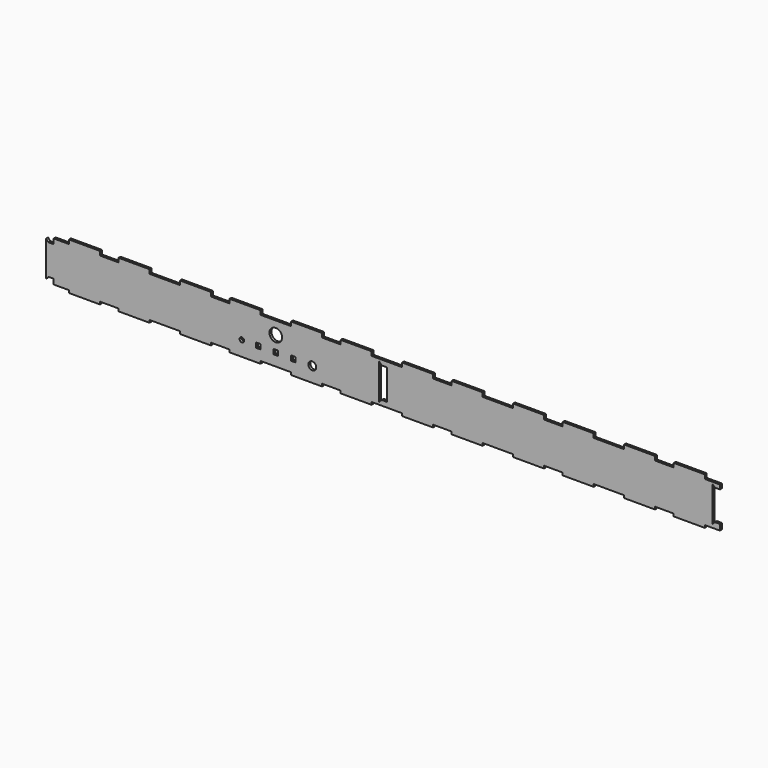
from build123d import *

# Parameters (mm, degrees)
F0_W      = 834.7400754492
F0_H      = 50.8
F1_DEPTH  = 3.048
F3_W      = 57.9247
F3_H      = 5.08
F3_W_2    = 115.8494
F3_H_2    = 3.1496
F4_DEPTH  = 3.048
F6_DEPTH  = 3.048
F7_DEPTH  = 3.049
F9_W      = 6.096
F9_H      = 6.096
F9_R      = 2.8702
F9_R_2    = 4.953
F9_R_3    = 7.9375
F10_DEPTH = 3.049
F11_DEPTH = 25.4
F12_W     = 38.1
F12_H     = 5.08
F12_H_2   = 3.1496
F13_DEPTH = 3.048


# Not quite as in the source:
# - a feature names something its author has since deleted; it is built from what else it names


with BuildPart() as f1:
    # F0 (on Front) → F1 (new body)
    with BuildSketch(Plane.XZ):
        with Locations((417.3700377246, 25.4)):
            Rectangle(F0_W, F0_H)
    extrude(amount=F1_DEPTH)

    # F3 (on face) → F4 (join)
    with BuildSketch(Plane.XZ.offset(3.048)):
        with Locations((28.96235, 53.34)):
            Rectangle(F3_W, F3_H)
        with Locations((139.1233459082, 53.34)):
            Rectangle(F3_W_2, F3_H)
        with Locations((278.2466918164, 53.34)):
            Rectangle(F3_W_2, F3_H)
        with Locations((417.3700377246, 53.34)):
            Rectangle(F3_W_2, F3_H)
        with Locations((556.4933836328, 53.34)):
            Rectangle(F3_W_2, F3_H)
        with Locations((695.616729541, 53.34)):
            Rectangle(F3_W_2, F3_H)
        with Locations((805.7777254492, 53.34)):
            Rectangle(F3_W, F3_H)
        with Locations((28.96235, -1.5748)):
            Rectangle(F3_W, F3_H_2)
        with Locations((139.1233459082, -1.5748)):
            Rectangle(F3_W_2, F3_H_2)
        with Locations((278.2466918164, -1.5748)):
            Rectangle(F3_W_2, F3_H_2)
        with Locations((417.3700377246, -1.5748)):
            Rectangle(F3_W_2, F3_H_2)
        with Locations((556.4933836328, -1.5748)):
            Rectangle(F3_W_2, F3_H_2)
        with Locations((695.616729541, -1.5748)):
            Rectangle(F3_W_2, F3_H_2)
        with Locations((805.7777254492, -1.5748)):
            Rectangle(F3_W, F3_H_2)
    extrude(amount=-F4_DEPTH)

    # F5 (on face) → F6 (join)
    with BuildSketch(Plane.XZ.offset(3.048)):
        Polygon((-6.35, 6.35), (0, 6.35), (0, 44.45), (-6.35, 44.45), (-9.525, 47.625), (-9.525, 3.175), align=None)
    extrude(amount=-F6_DEPTH)

    # F5 (on face) → F7 (cut, through all)
    with BuildSketch(Plane.XZ.offset(3.048)):
        Polygon((828.3900754492, 7.3152), (834.7400754492, 7.3152), (834.7400754492, 45.4152), (828.3900754492, 45.4152), (825.2150754492, 48.5902), (825.2150754492, 4.1402), align=None)
    extrude(amount=-F7_DEPTH, mode=Mode.SUBTRACT)

    # F9 (on face) → F10 (cut, through all)
    with BuildSketch(Plane.XZ.offset(3.048)):
        with Locations((256.3264918164, 15.621)):
            Rectangle(F9_W, F9_H)
        with Locations((278.2466918164, 15.621)):
            Rectangle(F9_W, F9_H)
        with Locations((300.1668918164, 15.621)):
            Rectangle(F9_W, F9_H)
        with Locations((235.7016918164, 15.621)):
            Circle(F9_R)
        with Locations((323.9666918164, 15.621)):
            Circle(F9_R_2)
        with Locations((278.2466918164, 34.671)):
            Circle(F9_R_3)
    extrude(amount=-F10_DEPTH, mode=Mode.SUBTRACT)

    # F8 (on face) → F11 (cut)
    with BuildSketch(Plane.XZ.offset(3.048)):
        Polygon((411.0200377246, 6.35), (417.3700377246, 6.35), (417.3700377246, 44.45), (411.0200377246, 44.45), (407.8450377246, 47.625), (407.8450377246, 3.175), align=None)
    extrude(amount=-F11_DEPTH, mode=Mode.SUBTRACT)

    # F12 (on face) → F13 (cut, through all)
    with BuildSketch(Plane.XZ.offset(3.048)):
        with Locations((139.1233459082, 53.34)):
            Rectangle(F12_W, F12_H)
        with Locations((278.2466918164, 53.34)):
            Rectangle(F12_W, F12_H)
        with Locations((417.3700377246, 53.34)):
            Rectangle(F12_W, F12_H)
        with Locations((556.4933836328, 53.34)):
            Rectangle(F12_W, F12_H)
        with Locations((695.616729541, 53.34)):
            Rectangle(F12_W, F12_H)
        with Locations((834.7400754492, 53.34)):
            Rectangle(F12_W, F12_H)
        with Locations((0, 53.34)):
            Rectangle(F12_W, F12_H)
        with Locations((0, -1.5748)):
            Rectangle(F12_W, F12_H_2)
        with Locations((139.1233459082, -1.5748)):
            Rectangle(F12_W, F12_H_2)
        with Locations((278.2466918164, -1.5748)):
            Rectangle(F12_W, F12_H_2)
        with Locations((417.3700377246, -1.5748)):
            Rectangle(F12_W, F12_H_2)
        with Locations((556.4933836328, -1.5748)):
            Rectangle(F12_W, F12_H_2)
        with Locations((695.616729541, -1.5748)):
            Rectangle(F12_W, F12_H_2)
        with Locations((834.7400754492, -1.5748)):
            Rectangle(F12_W, F12_H_2)
    extrude(amount=-F13_DEPTH, mode=Mode.SUBTRACT)


solid = f1.part
